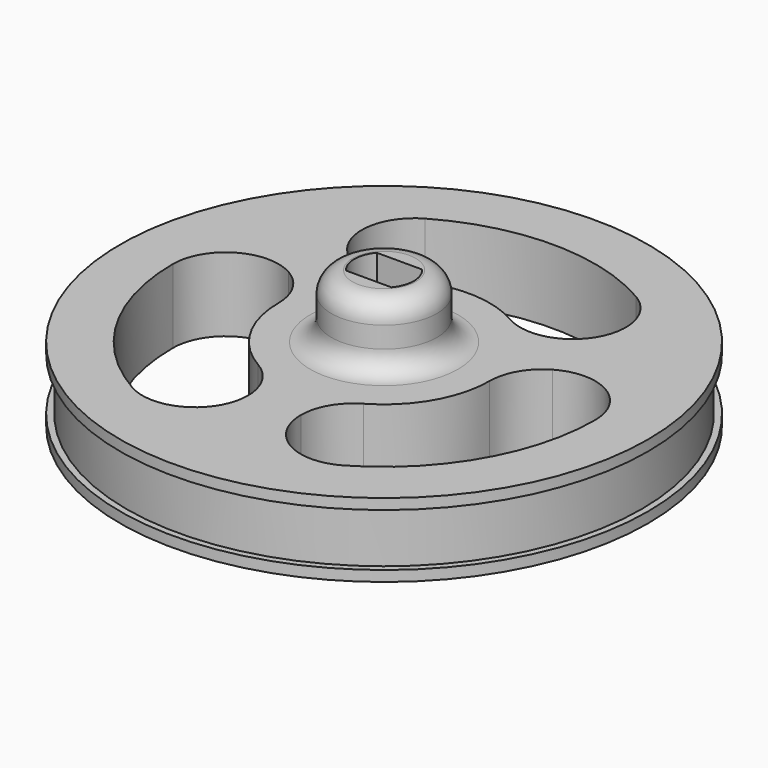
from build123d import *

# Parameters (mm, degrees)
F0_R         = 25
F1_DEPTH     = 7
F2_R         = 5
F3_DEPTH     = 6
F5_DEPTH     = 8
F7_R         = 25
F7_R_2       = 24.4
F8_DEPTH     = 5
F10_DEPTH    = 25
F11_R        = 5
F12_T1_DEPTH = 7
F13_R        = 2


# Not quite as in the source:
# - a fillet or chamfer that OpenCascade refuses, or shapes differently, is made with other operations: its cross-section is extruded or revolved along the edge and cut away or added


with BuildPart() as f1:
    # F0 (on Top) → F1 (new body)
    with BuildSketch(Plane.XY):
        Circle(F0_R)
    extrude(amount=F1_DEPTH)

    # F2 (on face) → F3 (join)
    with BuildSketch(Plane.XY.offset(7)):
        Circle(F2_R)
    extrude(amount=F3_DEPTH)

    # F4 (on face) → F5 (cut)
    with BuildSketch(Plane.XY.offset(13)):
        with BuildLine():
            Line((2.1498313887, 1.825), (-2.1498313887, 1.825))
            ThreePointArc((-2.1498313887, 1.825), (-2.82, 0), (-2.1498313887, -1.825))
            Line((-2.1498313887, -1.825), (2.1498313887, -1.825))
            ThreePointArc((2.1498313887, -1.825), (2.82, 0), (2.1498313887, 1.825))
        make_face()
    extrude(amount=-F5_DEPTH, mode=Mode.SUBTRACT)

    # F7 (on offset) → F8 (cut)
    with BuildSketch(Plane.XY.offset(1)):
        Circle(F7_R)
        Circle(F7_R_2, mode=Mode.SUBTRACT)
    extrude(amount=F8_DEPTH, mode=Mode.SUBTRACT)

    # F9 (on face) → F10 (cut)
    with BuildSketch(Plane.XY.offset(7)):
        with BuildLine():
            Line((7.1352549156, 7.0062926922), (15.9346604169, 12.0866318271))
            ThreePointArc((15.9346604169, 12.0866318271), (0, 20.0000017881), (-15.9346604169, 12.0866318271))
            Line((-15.9346604169, 12.0866318271), (-7.1352549156, 7.0062926922))
            ThreePointArc((-7.1352549156, 7.0062926922), (0, 10), (7.1352549156, 7.0062926922))
        make_face()
        with BuildLine():
            ThreePointArc((2.5, -19.8431366353), (15.0000012666, -13.2287578225), (20.0000017881, 0))
            ThreePointArc((20.0000017881, 0), (19.6047610649, 3.9564397015), (18.4346604169, 7.7565048082))
            Line((18.4346604169, 7.7565048082), (9.6352549156, 2.6761656733))
            ThreePointArc((9.6352549156, 2.6761656733), (9.9083941473, 1.3504537837), (10, 0))
            ThreePointArc((10, 0), (7.9056941504, -6.123724357), (2.5, -9.6824583655))
            Line((2.5, -9.6824583655), (2.5, -19.8431366353))
        make_face()
        with BuildLine():
            ThreePointArc((-18.4346604169, 7.7565048082), (-17.3205096243, -10.0000008941), (-2.5, -19.8431366353))
            Line((-2.5, -19.8431366353), (-2.5, -9.6824583655))
            ThreePointArc((-2.5, -9.6824583655), (-8.6602540378, -5), (-9.6352549156, 2.6761656733))
            Line((-9.6352549156, 2.6761656733), (-18.4346604169, 7.7565048082))
        make_face()
    extrude(amount=-F10_DEPTH, mode=Mode.SUBTRACT)

    # F11
    f11_edges = [f1.edges().sort_by_distance(p)[0] for p in [
        (-18.43466, 7.756505, 3.5),
        (-15.93466, 12.086632, 3.5),
        (15.93466, 12.086632, 3.5),
        (18.43466, 7.756505, 3.5),
        (2.5, -19.843137, 3.5),
        (-2.5, -19.843137, 3.5),
    ]]
    fillet(f11_edges, radius=F11_R)

    # F12: fillet of radius 5 on 6 edges, made by hand

    # F12_s2 → F12_t1 (join)
    with BuildSketch(Plane.XY):
        with BuildLine():
            ThreePointArc((-12.5, 4.3301270189), (-10.6698729811, 2.5), (-10, 0))
            ThreePointArc((-10, 0), (-9.9083941473, 1.3504537837), (-9.6352549156, 2.6761656733))
            Line((-9.6352549156, 2.6761656733), (-12.5, 4.3301270189))
        make_face()
        with BuildLine():
            ThreePointArc((-2.5, -12.9903810568), (-3.1698729811, -10.4903810568), (-5, -8.6602540378))
            ThreePointArc((-5, -8.6602540378), (-3.7846697903, -9.2561479341), (-2.5, -9.6824583655))
            Line((-2.5, -9.6824583655), (-2.5, -12.9903810568))
        make_face()
        with BuildLine():
            ThreePointArc((2.5, -12.9903810568), (3.1698729811, -10.4903810568), (5, -8.6602540378))
            ThreePointArc((5, -8.6602540378), (3.7846697903, -9.2561479341), (2.5, -9.6824583655))
            Line((2.5, -9.6824583655), (2.5, -12.9903810568))
        make_face()
        with BuildLine():
            ThreePointArc((12.5, 4.3301270189), (10.6698729811, 2.5), (10, 0))
            ThreePointArc((10, 0), (9.9083941473, 1.3504537837), (9.6352549156, 2.6761656733))
            Line((9.6352549156, 2.6761656733), (12.5, 4.3301270189))
        make_face()
        with BuildLine():
            ThreePointArc((10, 8.6602540378), (7.5, 7.9903810568), (5, 8.6602540378))
            ThreePointArc((5, 8.6602540378), (6.123724357, 7.9056941504), (7.1352549156, 7.0062926922))
            Line((7.1352549156, 7.0062926922), (10, 8.6602540378))
        make_face()
        with BuildLine():
            ThreePointArc((-10, 8.6602540378), (-7.5, 7.9903810568), (-5, 8.6602540378))
            ThreePointArc((-5, 8.6602540378), (-6.123724357, 7.9056941504), (-7.1352549156, 7.0062926922))
            Line((-7.1352549156, 7.0062926922), (-10, 8.6602540378))
        make_face()
    extrude(amount=F12_T1_DEPTH)

    # F13
    f13_edges = [f1.edges().sort_by_distance(p)[0] for p in [
        (-5, 0, 7),
        (-5, 0, 13),
    ]]
    fillet(f13_edges, radius=F13_R)


solid = f1.part
